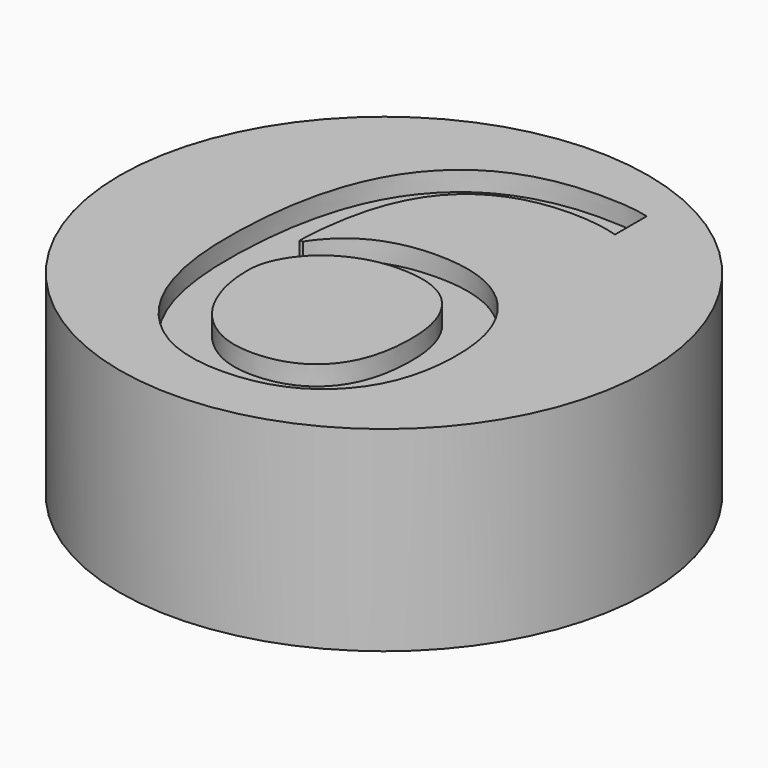
from build123d import *

# Parameters (mm, degrees)
F0_R         = 13.5
F1_DEPTH     = 10
F2_TEXT_SIZE = 29.0478649207
F3_DEPTH     = 1


# Not quite as in the source:
# - Text() gives the source's letters only with a copy of the font that has no kerning and outlines rounded to 1/6400 em; it was checked with that copy


with BuildPart() as f1:
    # F0 (on Top) → F1 (new body)
    with BuildSketch(Plane.XY):
        Circle(F0_R)
    extrude(amount=F1_DEPTH)

    # F2 (on face) → F3 (cut)
    with BuildSketch(Plane.XY.offset(10)):
        with Locations((-8.4599508423, -10.3940429915)):
            Text('6', F2_TEXT_SIZE, font='Open Sans', text_align=(TextAlign.LEFT, TextAlign.BOTTOM))
    extrude(amount=-F3_DEPTH, mode=Mode.SUBTRACT)


solid = f1.part
